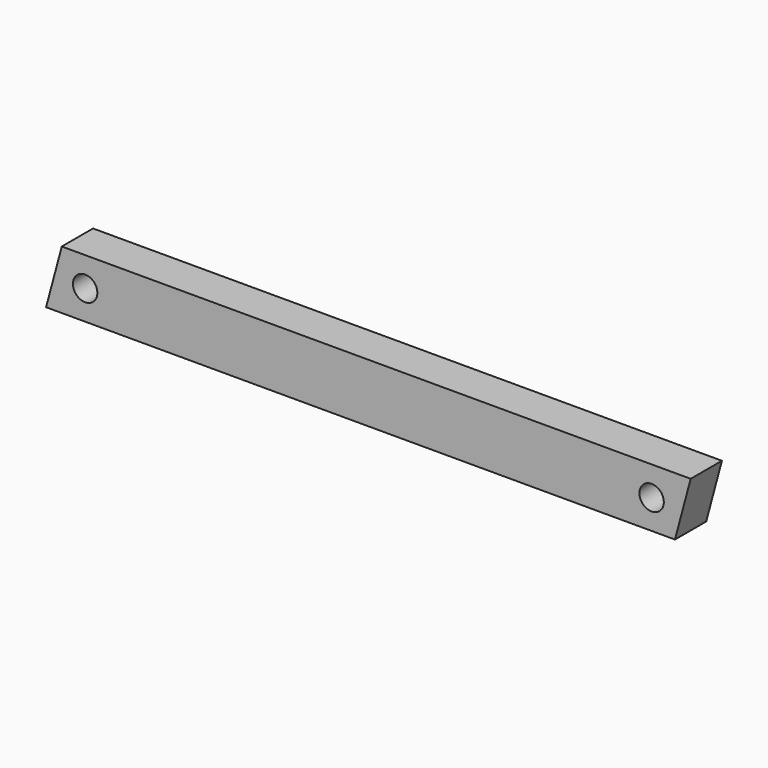
from build123d import *

# Parameters (mm, degrees)
F0_W     = 419.1
F0_H     = 38.1
F1_DEPTH = 25.4
F3_D     = 15.875
F5_DEPTH = 50.8
F7_DEPTH = 50.8


# Not quite as in the source:
# - a feature names something its author has since deleted; it is built from what else it names


with BuildPart() as f1:
    # F0 (on Front) → F1 (new body)
    with BuildSketch(Plane.XZ):
        with Locations((209.55, 19.05)):
            Rectangle(F0_W, F0_H)
    extrude(amount=F1_DEPTH)

    # F3 (through all)
    with Locations(Plane.XZ.offset(25.4)):
        with Locations((25.4, 19.05), (393.7, 19.05)):
            Hole(F3_D / 2)

    # F4 (on face) → F5 (cut)
    with BuildSketch(Plane.XZ.offset(25.4)):
        Polygon((0, 38.1), (0, 0), (10.2088642316, 38.1), align=None)
    extrude(amount=-F5_DEPTH, mode=Mode.SUBTRACT)

    # F6 (on face) → F7 (cut)
    with BuildSketch(Plane.XZ.offset(25.4)):
        Polygon((419.1, 0), (419.1, 38.1), (408.8911357684, 0), align=None)
    extrude(amount=-F7_DEPTH, mode=Mode.SUBTRACT)


solid = f1.part
